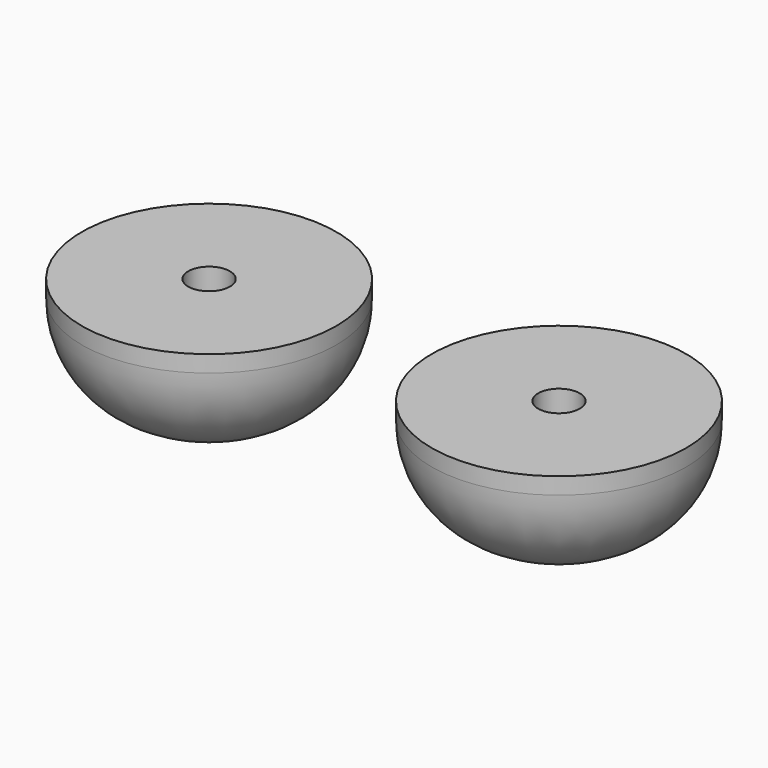
from build123d import *

# Parameters (mm, degrees)
F0_R     = 38.1
F0_R_2   = 6.2357
F1_DEPTH = 35
F2_R     = 30
F2_2_R   = 30
F3_DEPTH = 5


with BuildPart() as f1:
    # F0 (on Top) → F1 (new body)
    with BuildSketch(Plane.XY):
        with Locations((-52.0632453263, 30.500266701)):
            Circle(F0_R)
        with Locations((-52.0632453263, 30.500266701)):
            Circle(F0_R_2, mode=Mode.SUBTRACT)
    extrude(amount=F1_DEPTH)

    # F2
    f2_edges = [f1.edges().sort_by_distance(p)[0] for p in [
        (-90.163245, 30.500267, 0),
    ]]
    fillet(f2_edges, radius=F2_R)

    # F0 (on Top) → F3 (join)
    with BuildSketch(Plane.XY):
        with Locations((-52.0632453263, 30.500266701)):
            Circle(F0_R_2)
    extrude(amount=F3_DEPTH)


with BuildPart() as f1b:
    # F0 (on Top) → F1, piece 2 (new body)
    with BuildSketch(Plane.XY):
        with Locations((50.3609031439, 33.3374999464)):
            Circle(F0_R)
        with Locations((50.3609031439, 33.3374999464)):
            Circle(F0_R_2, mode=Mode.SUBTRACT)
    extrude(amount=F1_DEPTH)

    # F2#2
    f2_2_edges = [f1b.edges().sort_by_distance(p)[0] for p in [
        (12.260903, 33.3375, 0),
    ]]
    fillet(f2_2_edges, radius=F2_2_R)


with BuildPart() as f3:
    # F0 (on Top) → F3, piece 2 (new body)
    with BuildSketch(Plane.XY):
        with Locations((50.3609031439, 33.3374999464)):
            Circle(F0_R_2)
    extrude(amount=F3_DEPTH)


solid = Compound([f1.part, f1b.part, f3.part])
